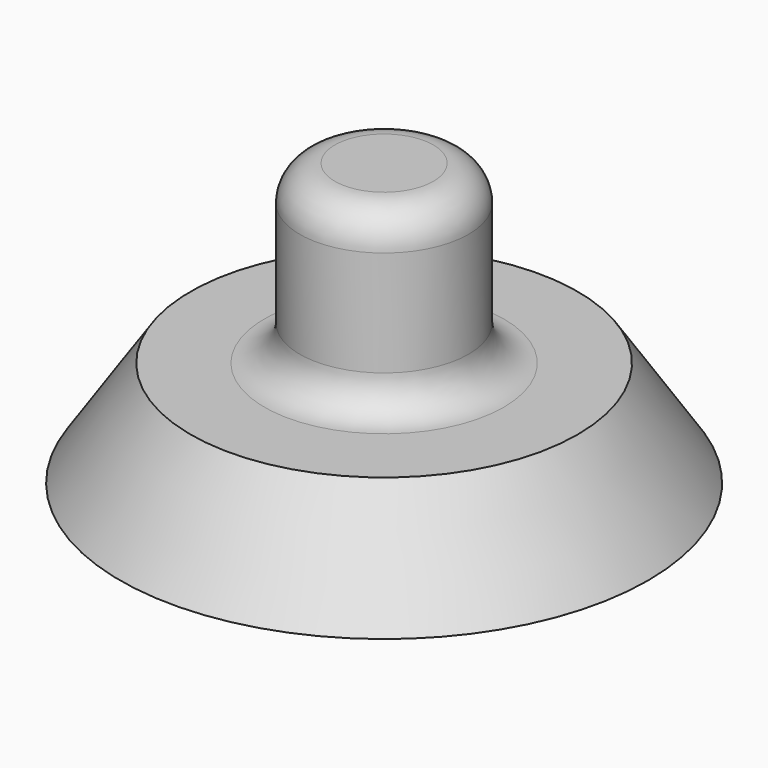
from build123d import *

# Parameters (mm, degrees)
F0_R     = 7.5
F1_DEPTH = 3
F2_SIZE2 = 2.99999
F2_SIZE  = 1.99999
F3_R     = 2.4
F4_DEPTH = 5
F5_R     = 1


# Not quite as in the source:
# - a fillet or chamfer is up to 0.001 mm smaller than in the source, because OpenCascade refuses the exact size


with BuildPart() as f1:
    # F0 (on Top) → F1 (new body)
    with BuildSketch(Plane.XY):
        Circle(F0_R)
    extrude(amount=F1_DEPTH)

    # F2 (size 2 and 3 in the source; OpenCascade refuses exactly that, so slightly less here)
    f2_edges = [f1.edges().sort_by_distance(p)[0] for p in [
        (-7.5, 0, 3),
    ]]
    f2_side = f1.faces().sort_by_distance((0, 0, 3))[0]
    chamfer(f2_edges, length=F2_SIZE, length2=F2_SIZE2, reference=f2_side)

    # F3 (on face) → F4 (join)
    with BuildSketch(Plane.XY.offset(3)):
        Circle(F3_R)
    extrude(amount=F4_DEPTH)

    # F5
    f5_edges = [f1.edges().sort_by_distance(p)[0] for p in [
        (-2.4, 0, 8),
        (-2.4, 0, 3),
    ]]
    fillet(f5_edges, radius=F5_R)


solid = f1.part
